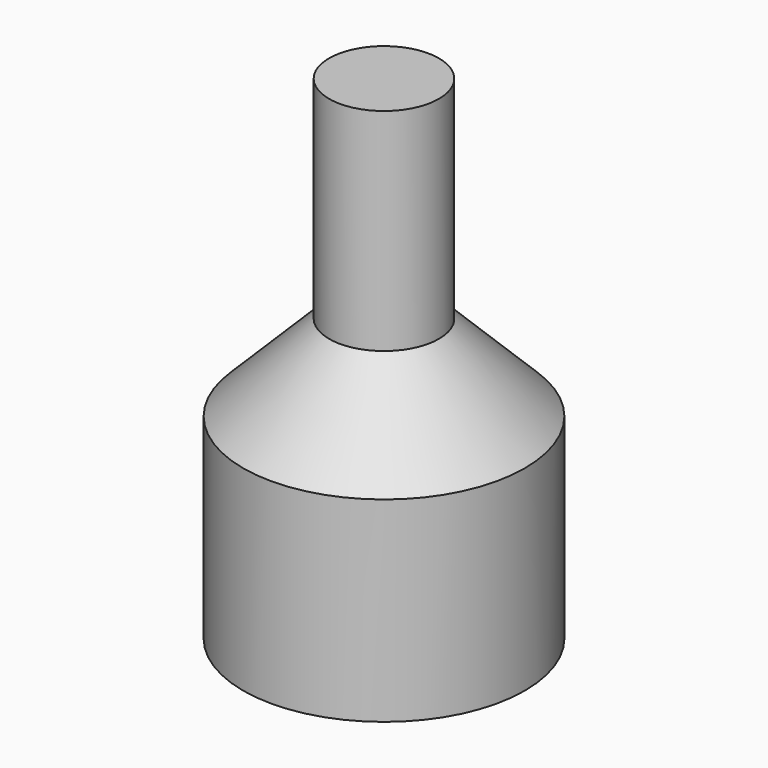
from build123d import *

# Parameters (mm, degrees)
F0_R        = 3.9
F1_DEPTH    = 15
F2_R        = 10
F3_DEPTH    = 20
F4_S5_R     = 3.9
F4_T6_DEPTH = 16


# Not quite as in the source:
# - a fillet or chamfer that OpenCascade refuses, or shapes differently, is made with other operations: its cross-section is extruded or revolved along the edge and cut away or added


with BuildPart() as f1:
    # F0 (on Top) → F1 (new body)
    with BuildSketch(Plane.XY):
        Circle(F0_R)
    extrude(amount=F1_DEPTH)

    # F2 (on Top) → F3 (join)
    with BuildSketch(Plane.XY):
        Circle(F2_R)
    extrude(amount=-F3_DEPTH)

    # F4: chamfer of 6.1 on 1 edges, made by hand


with BuildPart() as f4_tool2:
    # F4_s3 → F4_t4 (revolve)
    with BuildSketch(Plane.XZ):
        Polygon((10, -6.1), (3.9, 0), (10, 0), align=None)
    revolve(axis=Axis((0, 0, 0), (0, 0, 1)))

    # F4_s5 → F4_t6 (cut, symmetric)
    with BuildSketch(Plane.XY.offset(-3)):
        Circle(F4_S5_R)
    extrude(amount=F4_T6_DEPTH, both=True, mode=Mode.SUBTRACT)


with BuildPart() as f1_1:
    add(f1.part)

    # F4_t1: cut F4_tool2
    add(f4_tool2.part, mode=Mode.SUBTRACT)


solid = f1_1.part
